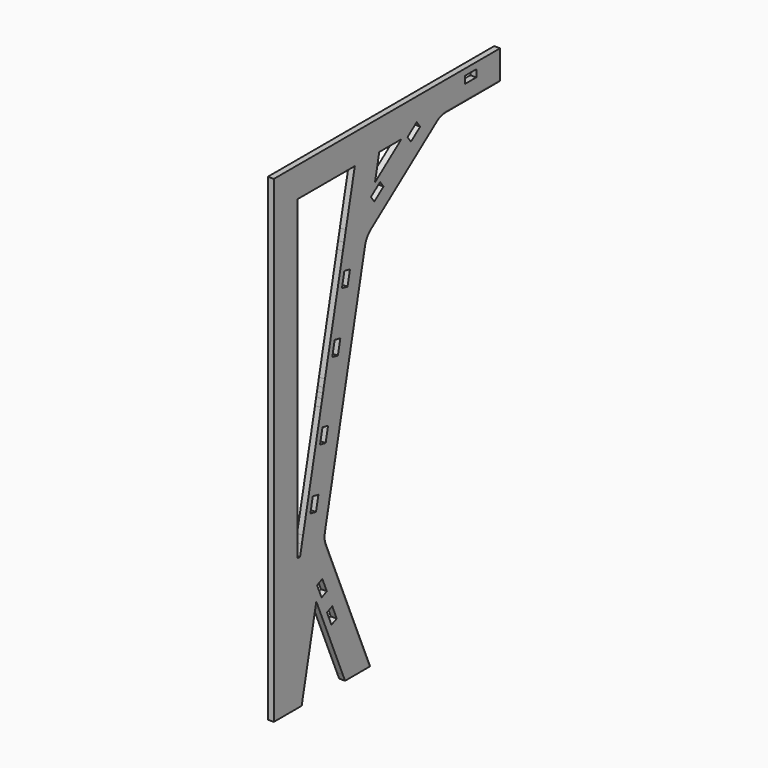
from build123d import *

# Parameters (mm, degrees)
F0_W     = 5.08
F0_H     = 2.54
F1_DEPTH = 2.1082
F2_R     = 0.762


with BuildPart() as f1:
    # F0 (on Right) → F1 (new body)
    with BuildSketch(Plane.YZ):
        with BuildLine():
            Line((0, 162.0091375), (0, 0))
            Line((0, 0), (12.335197777, 0))
            Line((12.335197777, 0), (18.8042013144, 29.896105485))
            Line((18.8042013144, 29.896105485), (30.5493542935, 2.3257501254))
            Line((30.5493542935, 2.3257501254), (31.5401391658, 0))
            Line((31.5401391658, 0), (31.5707651968, 0))
            Line((31.5707651968, 0), (40.8442968098, 0))
            Line((40.8442968098, 0), (20.5594925834, 47.616175108))
            Line((20.5594925834, 47.616175108), (39.5771112022, 135.5049402038))
            Line((39.5771112022, 135.5049402038), (73.5248959406, 160.7899383022))
            Line((73.5248959406, 160.7899383022), (100.203, 160.7899383022))
            Line((100.203, 160.7899383022), (100.203, 162.0091375))
            Line((100.203, 162.0091375), (82.1398573303, 162.0091375))
            ThreePointArc((82.1398573303, 162.0091375), (80.3438061061, 162.7530862758), (79.5998573303, 164.5491375))
            Line((79.5998573303, 164.5491375), (79.5998573303, 169.3418))
            Line((79.5998573303, 169.3418), (70.6874244764, 169.3418))
            Line((70.6874244764, 169.3418), (70.6874244764, 165.8480664454))
            Line((70.6874244764, 165.8480664454), (70.6874244764, 164.5491375))
            ThreePointArc((70.6874244764, 164.5491375), (70.0510915867, 162.8675752701), (68.4609272063, 162.0285589874))
            ThreePointArc((68.4609272063, 162.0285589874), (68.3044763435, 162.0139975214), (68.1474244764, 162.0091375))
            Line((68.1474244764, 162.0091375), (0, 162.0091375))
        make_face()
        Polygon((21.4843682503, 35.8535070154), (23.4753466245, 31.1799211209), (21.1385536773, 30.1844319338), (19.147575303, 34.8580178283), align=None, mode=Mode.SUBTRACT)
        Polygon((25.8665425285, 25.5668719827), (27.8575209028, 20.8932860882), (25.5207279555, 19.8977969011), (23.5297495813, 24.5713827956), align=None, mode=Mode.SUBTRACT)
        with BuildLine():
            Line((12.3986134924, 50.3752630702), (11.6175919588, 46.7658196656))
            Line((11.6175919588, 46.7658196656), (10.5918, 46.7658196656))
            Line((10.5918, 46.7658196656), (10.5918, 158.7579375))
            Line((10.5918, 158.7579375), (35.8507619547, 158.7579375))
            Line((35.8507619547, 158.7579375), (31.8897708968, 140.4524587956))
            Line((31.8897708968, 140.4524587956), (31.1087493632, 136.8430153909))
            Line((31.1087493632, 136.8430153909), (35.5475592049, 135.882533211))
            ThreePointArc((35.5475592049, 135.882533211), (37.1456481821, 134.7755682604), (37.4929253116, 132.8628062845))
            Line((37.4929253116, 132.8628062845), (29.5595533377, 96.1992113407))
            ThreePointArc((29.5595533377, 96.1992113407), (28.452588387, 94.6011223635), (26.5398264112, 94.2538452339))
            Line((26.5398264112, 94.2538452339), (22.1010165695, 95.2143274138))
            Line((22.1010165695, 95.2143274138), (21.7536814278, 93.6091392306))
            Line((21.7536814278, 93.6091392306), (21.4063462861, 92.0039510473))
            Line((21.4063462861, 92.0039510473), (25.8451561277, 91.0434688674))
            ThreePointArc((25.8451561277, 91.0434688674), (27.4432451049, 89.9365039168), (27.7905222345, 88.0237419409))
            Line((27.7905222345, 88.0237419409), (19.8571502605, 51.3601469971))
            ThreePointArc((19.8571502605, 51.3601469971), (18.7501853099, 49.7620580199), (16.837423334, 49.4147808903))
            Line((16.837423334, 49.4147808903), (12.3986134924, 50.3752630702))
        make_face(mode=Mode.SUBTRACT)
        Polygon((47.0613097153, 149.2568137468), (48.5785484084, 147.2197602993), (44.5044415132, 144.1852829132), (42.9872028202, 146.2223363607), align=None, mode=Mode.SUBTRACT)
        Polygon((44.8088104432, 150.074821282), (46.6876875952, 158.7579375), (56.4668125154, 158.7579375), align=None, mode=Mode.SUBTRACT)
        Polygon((63.2751536106, 161.3332132886), (64.7923923036, 159.296159841), (60.7182854085, 156.2616824549), (59.2010467154, 158.2987359025), align=None, mode=Mode.SUBTRACT)
        with BuildLine():
            Line((0, 164.5491375), (0, 162.0091375))
            Line((0, 162.0091375), (68.1474244764, 162.0091375))
            ThreePointArc((68.1474244764, 162.0091375), (68.3044763435, 162.0139975214), (68.4609272063, 162.0285589874))
            Line((68.4609272063, 162.0285589874), (69.6856973646, 162.9407926238))
            Line((69.6856973646, 162.9407926238), (68.1474244764, 165.0060867035))
            Line((68.1474244764, 165.0060867035), (68.1474244764, 164.5491375))
            Line((68.1474244764, 164.5491375), (55.1748093832, 164.5491375))
            Line((55.1748093832, 164.5491375), (50.0948093832, 164.5491375))
            Line((50.0948093832, 164.5491375), (10.3999171089, 164.5491375))
            Line((10.3999171089, 164.5491375), (5.3199171089, 164.5491375))
            Line((5.3199171089, 164.5491375), (0, 164.5491375))
        make_face()
        Polygon((0, 169.3418), (0, 164.5491375), (5.3199171089, 164.5491375), (5.3199171089, 167.0891375), (10.3999171089, 167.0891375), (10.3999171089, 164.5491375), (50.0948093832, 164.5491375), (50.0948093832, 167.0891375), (55.1748093832, 167.0891375), (55.1748093832, 164.5491375), (68.1474244764, 164.5491375), (68.1474244764, 165.0060867035), (68.1474244764, 169.3418), align=None)
        with Locations((7.8599171089, 165.8191375)):
            Rectangle(F0_W, F0_H)
        with BuildLine():
            Line((69.6856973646, 162.9407926238), (68.4609272063, 162.0285589874))
            ThreePointArc((68.4609272063, 162.0285589874), (70.0510915867, 162.8675752701), (70.6874244764, 164.5491375))
            Line((70.6874244764, 164.5491375), (70.6874244764, 165.8480664454))
            Line((70.6874244764, 165.8480664454), (70.6874244764, 169.3418))
            Line((70.6874244764, 169.3418), (68.1474244764, 169.3418))
            Line((68.1474244764, 169.3418), (68.1474244764, 165.0060867035))
            Line((68.1474244764, 165.0060867035), (69.6856973646, 162.9407926238))
        make_face()
        with Locations((52.6348093832, 165.8191375)):
            Rectangle(F0_W, F0_H)
        with BuildLine():
            Line((20.5594925834, 47.616175108), (40.8442968098, 0))
            Line((40.8442968098, 0), (43.053, 0))
            Line((43.053, 0), (23.4736756901, 45.9601445708))
            ThreePointArc((23.4736756901, 45.9601445708), (22.9941781878, 47.847708452), (23.1092917667, 49.7918185633))
            Line((23.1092917667, 49.7918185633), (40.8984089502, 132.0031391675))
            ThreePointArc((40.8984089502, 132.0031391675), (41.765080018, 134.0967787378), (43.3116785091, 135.7528217618))
            Line((43.3116785091, 135.7528217618), (72.5103326221, 157.500571119))
            ThreePointArc((72.5103326221, 157.500571119), (74.3053957564, 158.4354047741), (76.3034293547, 158.7579375))
            Line((76.3034293547, 158.7579375), (100.203, 158.7579375))
            Line((100.203, 158.7579375), (100.203, 160.7899383022))
            Line((100.203, 160.7899383022), (73.5248959406, 160.7899383022))
            Line((73.5248959406, 160.7899383022), (39.5771112022, 135.5049402038))
            Line((39.5771112022, 135.5049402038), (20.5594925834, 47.616175108))
        make_face()
        with BuildLine():
            Line((82.1398573303, 169.3418), (79.5998573303, 169.3418))
            Line((79.5998573303, 169.3418), (79.5998573303, 164.5491375))
            ThreePointArc((79.5998573303, 164.5491375), (80.3438061061, 162.7530862758), (82.1398573303, 162.0091375))
            Line((82.1398573303, 162.0091375), (100.203, 162.0091375))
            Line((100.203, 162.0091375), (100.203, 164.5491375))
            Line((100.203, 164.5491375), (89.6502663064, 164.5491375))
            Line((89.6502663064, 164.5491375), (84.5702663064, 164.5491375))
            Line((84.5702663064, 164.5491375), (82.1398573303, 164.5491375))
            Line((82.1398573303, 164.5491375), (82.1398573303, 169.3418))
        make_face()
        Polygon((100.203, 169.3418), (82.1398573303, 169.3418), (82.1398573303, 164.5491375), (84.5702663064, 164.5491375), (84.5702663064, 167.0891375), (89.6502663064, 167.0891375), (89.6502663064, 164.5491375), (100.203, 164.5491375), align=None)
        with BuildLine():
            Line((12.9357939022, 52.8578095868), (12.3986134924, 50.3752630702))
            Line((12.3986134924, 50.3752630702), (16.837423334, 49.4147808903))
            ThreePointArc((16.837423334, 49.4147808903), (18.7501853099, 49.7620580199), (19.8571502605, 51.3601469971))
            Line((19.8571502605, 51.3601469971), (27.7905222345, 88.0237419409))
            ThreePointArc((27.7905222345, 88.0237419409), (27.4432451049, 89.9365039168), (25.8451561277, 91.0434688674))
            Line((25.8451561277, 91.0434688674), (21.4063462861, 92.0039510473))
            Line((21.4063462861, 92.0039510473), (20.8691658762, 89.5214045307))
            Line((20.8691658762, 89.5214045307), (25.3079757178, 88.5609223508))
            Line((25.3079757178, 88.5609223508), (24.0175885553, 82.5974767434))
            Line((24.0175885553, 82.5974767434), (22.9432277355, 77.6323837102))
            Line((22.9432277355, 77.6323837102), (19.7419229759, 62.8377489213))
            Line((19.7419229759, 62.8377489213), (18.6675621562, 57.872655888))
            Line((18.6675621562, 57.872655888), (17.3746037439, 51.8973274069))
            Line((17.3746037439, 51.8973274069), (12.9357939022, 52.8578095868))
        make_face()
        Polygon((20.8691658762, 89.5214045307), (12.9357939022, 52.8578095868), (17.3746037439, 51.8973274069), (18.6675621562, 57.872655888), (16.1850156395, 58.4098362979), (17.2593764593, 63.3749293312), (19.7419229759, 62.8377489213), (22.9432277355, 77.6323837102), (20.4606812189, 78.16956412), (21.5350420386, 83.1346571533), (24.0175885553, 82.5974767434), (25.3079757178, 88.5609223508), align=None)
        with BuildLine():
            Line((35.5475592049, 135.882533211), (31.1087493632, 136.8430153909))
            Line((31.1087493632, 136.8430153909), (30.5715689534, 134.3604688743))
            Line((30.5715689534, 134.3604688743), (35.010378795, 133.3999866944))
            Line((35.010378795, 133.3999866944), (33.7174203827, 127.4246582133))
            Line((33.7174203827, 127.4246582133), (32.643059563, 122.45956518))
            Line((32.643059563, 122.45956518), (29.4417548033, 107.6649303911))
            Line((29.4417548033, 107.6649303911), (28.3673939836, 102.6998373579))
            Line((28.3673939836, 102.6998373579), (27.077006821, 96.7363917505))
            Line((27.077006821, 96.7363917505), (22.6381969794, 97.6968739305))
            Line((22.6381969794, 97.6968739305), (22.1010165695, 95.2143274138))
            Line((22.1010165695, 95.2143274138), (26.5398264112, 94.2538452339))
            ThreePointArc((26.5398264112, 94.2538452339), (28.452588387, 94.6011223635), (29.5595533377, 96.1992113407))
            Line((29.5595533377, 96.1992113407), (37.4929253116, 132.8628062845))
            ThreePointArc((37.4929253116, 132.8628062845), (37.1456481821, 134.7755682604), (35.5475592049, 135.882533211))
        make_face()
        Polygon((35.010378795, 133.3999866944), (30.5715689534, 134.3604688743), (22.6381969794, 97.6968739305), (27.077006821, 96.7363917505), (28.3673939836, 102.6998373579), (25.884847467, 103.2370177677), (26.9592082867, 108.202110801), (29.4417548033, 107.6649303911), (32.643059563, 122.45956518), (30.1605130463, 122.9967455899), (31.2348738661, 127.9618386231), (33.7174203827, 127.4246582133), align=None)
    extrude(amount=F1_DEPTH)

    # F2
    f2_edges = [f1.edges().sort_by_distance(p)[0] for p in [
        (2.1082, 32.00385, 90.897479),
        (2.1082, 33.263338, 22.980072),
        (2.1082, 22.994178, 47.847708),
        (2.1082, 41.76508, 134.096779),
        (2.1082, 57.911006, 146.626696),
        (2.1082, 74.305396, 158.435405),
        (2.1082, 88.253215, 158.757937),
    ]]
    fillet(f2_edges, radius=F2_R)


solid = f1.part
